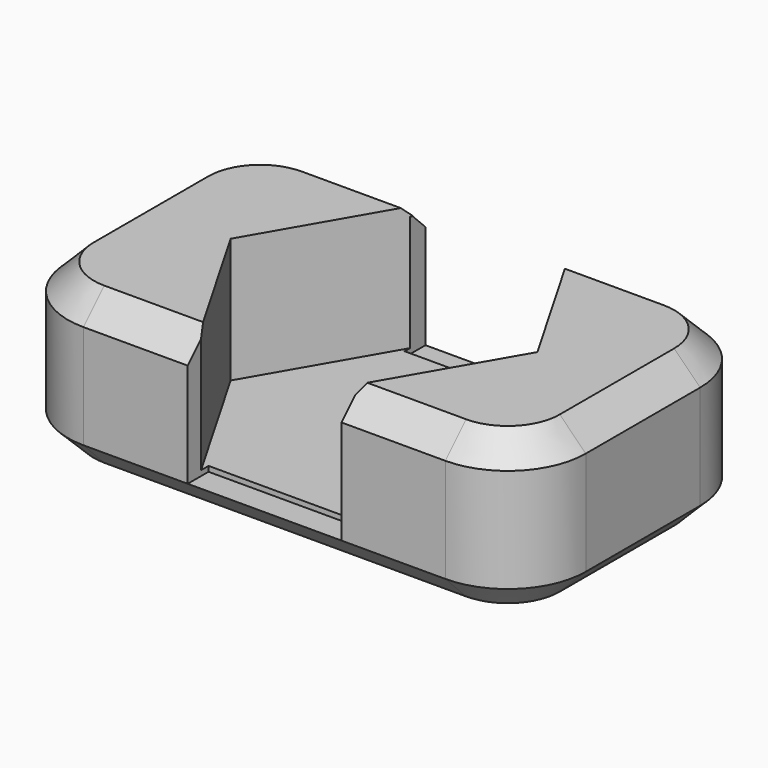
from build123d import *

# Parameters (mm, degrees)
F1_DEPTH     = 6
F3_DEPTH     = 4.8
F4_T1_DEPTH  = 13.92
F4_T3_DEPTH  = 5.5
F4_T6_ANGLE  = 90
F4_T8_ANGLE  = 90
F4_T10_ANGLE = 90
F4_T12_ANGLE = 90
F4_T14_ANGLE = 90
F4_T16_ANGLE = 90
F4_T18_ANGLE = 90
F4_T20_ANGLE = 90
F5_W         = 5.9125532862
F5_H         = 4.6649316102
F6_DEPTH     = 1
F7_W         = 5.9137202334
F7_H         = 4.6533403695
F8_DEPTH     = 1


# Not quite as in the source:
# - a fillet or chamfer that OpenCascade refuses, or shapes differently, is made with other operations: its cross-section is extruded or revolved along the edge and cut away or added


with BuildPart() as f1:
    # F0 (on Top) → F1 (new body)
    with BuildSketch(Plane.XY):
        with BuildLine():
            Line((6.96, 5.75), (-6.96, 5.75))
            ThreePointArc((-6.96, 5.75), (-9.0813203436, 4.8713203436), (-9.96, 2.75))
            Line((-9.96, 2.75), (-9.96, -2.75))
            ThreePointArc((-9.96, -2.75), (-9.0813203436, -4.8713203436), (-6.96, -5.75))
            Line((-6.96, -5.75), (6.96, -5.75))
            ThreePointArc((6.96, -5.75), (9.0813203436, -4.8713203436), (9.96, -2.75))
            Line((9.96, -2.75), (9.96, 2.75))
            ThreePointArc((9.96, 2.75), (9.0813203436, 4.8713203436), (6.96, 5.75))
        make_face()
    extrude(amount=F1_DEPTH)

    # F2 (on face) → F3 (cut)
    with BuildSketch(Plane.XY.offset(6)):
        Polygon((2.95, 5.1095498823), (-2.95, 5.1095498823), (-5.9, 0), (-2.95, -5.1095498823), (2.95, -5.1095498823), (5.9, 0), align=None)
    extrude(amount=-F3_DEPTH, mode=Mode.SUBTRACT)

    # F4: chamfer of 1 on 2 edges, made by hand

    # F4_s2 → F4_t1 (cut)
    with BuildSketch(Plane.YZ.offset(-6.96)):
        Polygon((5.75, 5), (4.75, 6), (5.75, 6), align=None)
        Polygon((5.75, 1), (4.75, 0), (5.75, 0), align=None)
        Polygon((-4.75, 0), (-5.75, 1), (-5.75, 0), align=None)
        Polygon((-4.75, 6), (-5.75, 5), (-5.75, 6), align=None)
    extrude(amount=F4_T1_DEPTH, mode=Mode.SUBTRACT)

    # F4_s4 → F4_t3 (cut)
    with BuildSketch(Plane.XZ.offset(-2.75)):
        Polygon((-8.96, 0), (-9.96, 1), (-9.96, 0), align=None)
        Polygon((8.96, 0), (9.96, 1), (9.96, 0), align=None)
        Polygon((-8.96, 6), (-9.96, 5), (-9.96, 6), align=None)
        Polygon((8.96, 6), (9.96, 5), (9.96, 6), align=None)
    extrude(amount=F4_T3_DEPTH, mode=Mode.SUBTRACT)

    # F4_s5 → F4_t6 (revolve, cut)
    with BuildSketch(Plane.XZ.offset(-2.75)):
        Polygon((9.96, 1), (8.96, 0), (9.96, 0), align=None)
    revolve(axis=Axis((6.96, 2.75, 0), (0, 0, 1)), revolution_arc=F4_T6_ANGLE, mode=Mode.SUBTRACT)

    # F4_s7 → F4_t8 (revolve, cut)
    with BuildSketch(Plane.YZ.offset(-6.96)):
        Polygon((5.75, 1), (4.75, 0), (5.75, 0), align=None)
    revolve(axis=Axis((-6.96, 2.75, 0), (0, 0, 1)), revolution_arc=F4_T8_ANGLE, mode=Mode.SUBTRACT)

    # F4_s9 → F4_t10 (revolve, cut)
    with BuildSketch(Plane.XZ.offset(2.75)):
        Polygon((-8.96, 0), (-9.96, 1), (-9.96, 0), align=None)
    revolve(axis=Axis((-6.96, -2.75, 0), (0, 0, 1)), revolution_arc=F4_T10_ANGLE, mode=Mode.SUBTRACT)

    # F4_s11 → F4_t12 (revolve, cut)
    with BuildSketch(Plane.YZ.offset(6.96)):
        Polygon((-4.75, 0), (-5.75, 1), (-5.75, 0), align=None)
    revolve(axis=Axis((6.96, -2.75, 0), (0, 0, 1)), revolution_arc=F4_T12_ANGLE, mode=Mode.SUBTRACT)

    # F4_s13 → F4_t14 (revolve, cut)
    with BuildSketch(Plane.XZ.offset(-2.75)):
        Polygon((9.96, 5), (8.96, 6), (9.96, 6), align=None)
    revolve(axis=Axis((6.96, 2.75, 6), (0, 0, 1)), revolution_arc=F4_T14_ANGLE, mode=Mode.SUBTRACT)

    # F4_s15 → F4_t16 (revolve, cut)
    with BuildSketch(Plane.YZ.offset(-6.96)):
        Polygon((5.75, 5), (4.75, 6), (5.75, 6), align=None)
    revolve(axis=Axis((-6.96, 2.75, 6), (0, 0, 1)), revolution_arc=F4_T16_ANGLE, mode=Mode.SUBTRACT)

    # F4_s17 → F4_t18 (revolve, cut)
    with BuildSketch(Plane.XZ.offset(2.75)):
        Polygon((-8.96, 6), (-9.96, 5), (-9.96, 6), align=None)
    revolve(axis=Axis((-6.96, -2.75, 6), (0, 0, 1)), revolution_arc=F4_T18_ANGLE, mode=Mode.SUBTRACT)

    # F4_s19 → F4_t20 (revolve, cut)
    with BuildSketch(Plane.YZ.offset(6.96)):
        Polygon((-4.75, 6), (-5.75, 5), (-5.75, 6), align=None)
    revolve(axis=Axis((6.96, -2.75, 6), (0, 0, 1)), revolution_arc=F4_T20_ANGLE, mode=Mode.SUBTRACT)

    # F5 (on face) → F6 (cut)
    with BuildSketch(Plane.XZ.offset(5.75)):
        with Locations((0.007480965, 3.3324658051)):
            Rectangle(F5_W, F5_H)
    extrude(amount=-F6_DEPTH, mode=Mode.SUBTRACT)

    # F7 (on face) → F8 (cut)
    with BuildSketch(Plane(origin=(0, 5.75, 0), x_dir=(-1, 0, 0), z_dir=(0, 1, 0))):
        with Locations((0.0472323736, 3.3266701847)):
            Rectangle(F7_W, F7_H)
    extrude(amount=-F8_DEPTH, mode=Mode.SUBTRACT)


solid = f1.part
